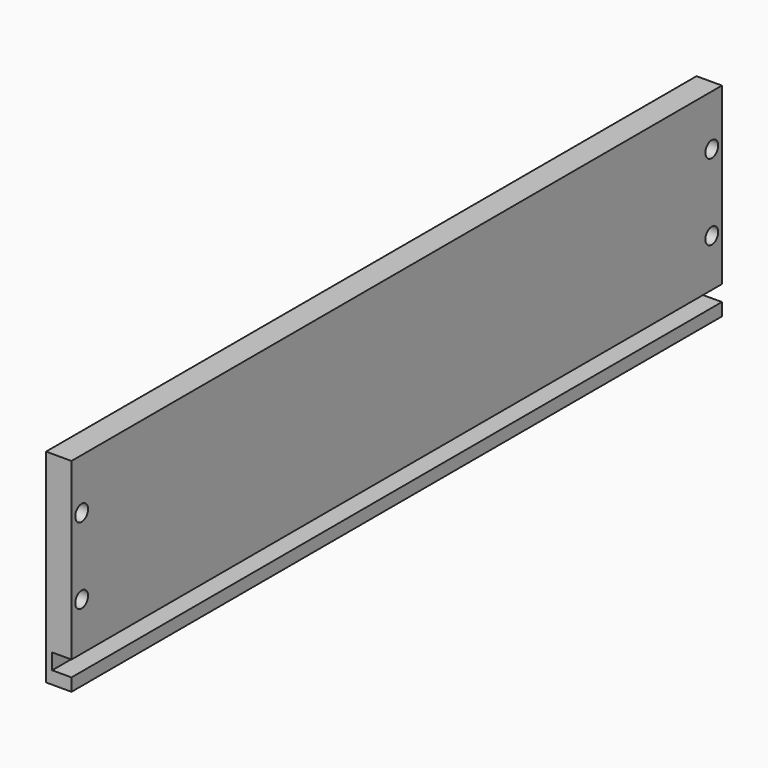
from build123d import *

# Parameters (mm, degrees)
F0_W     = 406.4
F0_H     = 101.6
F1_DEPTH = 12.7
F2_W     = 406.4
F2_H     = 7.874
F3_DEPTH = 9.652
F5_D     = 8.001
F5_DEPTH = 9.652
F5_TIP   = 2.4037429064


with BuildPart() as f1:
    # F0 (on Right) → F1 (new body)
    with BuildSketch(Plane.YZ):
        Rectangle(F0_W, F0_H)
    extrude(amount=F1_DEPTH)

    # F2 (on face) → F3 (cut)
    with BuildSketch(Plane.YZ.offset(12.7)):
        with Locations((0, -40.513)):
            Rectangle(F2_W, F2_H)
    extrude(amount=-F3_DEPTH, mode=Mode.SUBTRACT)

    # F5
    with Locations(Plane.YZ.offset(12.7)):
        with Locations((-196.85, 25.4), (-196.85, -12.7), (196.85, 25.4), (196.85, -12.7)):
            Hole(F5_D / 2, depth=F5_DEPTH)
            with Locations((0, 0, -(F5_DEPTH + F5_TIP / 2))):  # 118° drill point
                Cone(0, F5_D / 2, F5_TIP, mode=Mode.SUBTRACT)


solid = f1.part
